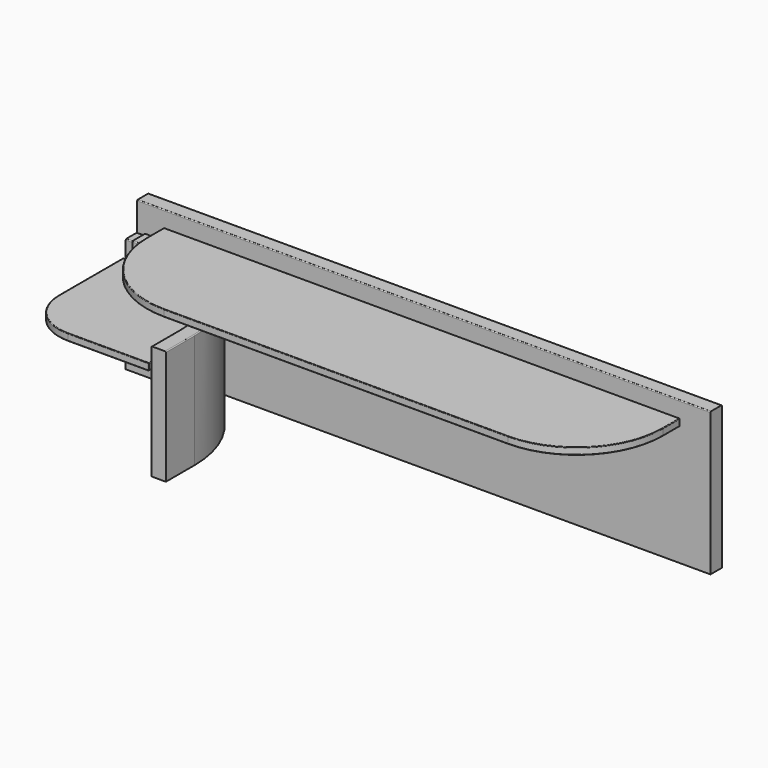
from build123d import *

# Parameters (mm, degrees)
F0_W                      = 2000
F0_H                      = 50
F1_DEPTH                  = 500
F4_DEPTH                  = 24
F5_R                      = 3
F6_R                      = 2
F8_DEPTH                  = 400
F11_DEPTH                 = 35
F13_DEPTH                 = 24
F14_R                     = 7.5
F15_DEPTH                 = 10
DRAFT_F15_DRAFTED_ANGLE   = 45
DRAFT_F15_2_DRAFTED_ANGLE = 45
F16_R                     = 5
F17_DEPTH                 = 6
F18_R                     = 3.5
F19_DEPTH                 = 25
F20_R                     = 3
F21_R                     = 2


# Not quite as in the source:
# - an extrude with a draft is written as a straight extrude whose walls are then drafted


with BuildPart() as f1:
    # F0 (on Top) → F1 (new body)
    with BuildSketch(Plane.XY):
        with Locations((1000, 25)):
            Rectangle(F0_W, F0_H)
    extrude(amount=F1_DEPTH)

    # F5
    f5_edges = [f1.edges().sort_by_distance(p)[0] for p in [
        (1000, 0, 500),
        (1000, 50, 500),
    ]]
    fillet(f5_edges, radius=F5_R)


with BuildPart() as f4:
    # F3 (on offset) → F4 (new body)
    with BuildSketch(Plane.XY.offset(426)):
        with BuildLine():
            Line((1900, -8), (100, -8))
            Line((100, -8), (100, -83))
            ThreePointArc((100, -83), (187.867965644, -295.132034356), (400, -383))
            Line((400, -383), (1600, -383))
            ThreePointArc((1600, -383), (1812.132034356, -295.132034356), (1900, -83))
            Line((1900, -83), (1900, -8))
        make_face()
    extrude(amount=F4_DEPTH)

    # F6
    f6_edges = [f4.edges().sort_by_distance(p)[0] for p in [
        (100, -45.5, 450),
        (187.867966, -295.132034, 450),
        (1000, -383, 426),
        (100, -8, 438),
        (1000, -8, 450),
        (1000, -8, 426),
        (1900, -8, 438),
    ]]
    fillet(f6_edges, radius=F6_R)


with BuildPart() as f8:
    # F7 (on Top) → F8 (new body)
    with BuildSketch(Plane.XY):
        with BuildLine():
            Line((125, 0), (0, 0))
            Line((0, 0), (0, -50))
            Line((0, -50), (125, -50))
            ThreePointArc((125, -50), (354.8097038856, -145.1902961144), (450, -375))
            Line((450, -375), (450, -500))
            Line((450, -500), (500, -500))
            Line((500, -500), (500, -375))
            ThreePointArc((500, -375), (390.165042945, -109.834957055), (125, 0))
        make_face()
    extrude(amount=F8_DEPTH)

    # F20
    f20_edges = [f8.edges().sort_by_distance(p)[0] for p in [
        (354.809704, -145.190296, 400),
        (62.5, 0, 400),
        (450, -437.5, 400),
        (500, -437.5, 400),
        (390.165043, -109.834957, 400),
        (62.5, -50, 400),
    ]]
    fillet(f20_edges, radius=F20_R)


with BuildPart() as f11:
    # F10 (on offset) → F11 (new body, symmetric)
    with BuildSketch(Plane(origin=(62.5, 0, 0), x_dir=(0, -1, 0), z_dir=(-1, 0, 0))):
        with BuildLine():
            ThreePointArc((50, 319), (50.8786796564, 316.8786796564), (53, 316))
            Line((53, 316), (104, 316))
            ThreePointArc((104, 316), (104.7071067812, 316.2928932188), (105, 317))
            Line((105, 317), (105, 320))
            ThreePointArc((105, 320), (104.7071067812, 320.7071067812), (104, 321))
            Line((104, 321), (58, 321))
            ThreePointArc((58, 321), (55.8786796564, 321.8786796564), (55, 324))
            Line((55, 324), (55, 402))
            ThreePointArc((55, 402), (54.1213203436, 404.1213203436), (52, 405))
            Line((52, 405), (-2, 405))
            ThreePointArc((-2, 405), (-4.1213203436, 404.1213203436), (-5, 402))
            Line((-5, 402), (-5, 355))
            ThreePointArc((-5, 355), (-1.4644660941, 353.5355339059), (0, 350))
            Line((0, 350), (0, 397))
            ThreePointArc((0, 397), (0.8786796564, 399.1213203436), (3, 400))
            Line((3, 400), (47, 400))
            ThreePointArc((47, 400), (49.1213203436, 399.1213203436), (50, 397))
            Line((50, 397), (50, 319))
        make_face()
        with BuildLine():
            ThreePointArc((-5, 345), (-1.4644660941, 346.4644660941), (0, 350))
            ThreePointArc((0, 350), (-1.4644660941, 353.5355339059), (-5, 355))
            Line((-5, 355), (-5, 345))
        make_face()
        with BuildLine():
            ThreePointArc((-5, 355), (-10, 350), (-5, 345))
            Line((-5, 345), (-5, 355))
        make_face()
    extrude(amount=F11_DEPTH, both=True)


with BuildPart() as f13:
    # F12 (on face) → F13 (new body)
    with BuildSketch(Plane.XY.offset(321)):
        with BuildLine():
            Line((125, -60), (-1.2988302449, -60))
            Line((-1.2988302449, -60), (-1.2988302449, -340))
            ThreePointArc((-1.2988302449, -340), (45.5640847653, -453.1370849898), (158.7011697551, -500))
            Line((158.7011697551, -500), (440, -500))
            Line((440, -500), (440, -375))
            ThreePointArc((440, -375), (347.7386360738, -152.2613639262), (125, -60))
        make_face()
    extrude(amount=F13_DEPTH)


with BuildPart() as f15_drafted:
    # F14 (on face) → F15 (new body)
    with BuildSketch(Plane(origin=(0, 0, 316), x_dir=(1, 0, 0), z_dir=(0, 0, -1))):
        with Locations((47.5, 82)):
            Circle(F14_R)
    extrude(amount=-F15_DEPTH)

    # draft_F15_drafted
    draft_f15_drafted_walls = [f15_drafted.faces().sort_by_distance(p)[0] for p in [
        (40, -82, 322.6666666667),
    ]]
    draft(draft_f15_drafted_walls, neutral_plane=Plane.XY.offset(316), angle=DRAFT_F15_DRAFTED_ANGLE)


with BuildPart() as f11_1:
    add(f11.part)

    # join_F15_drafted: cut F15_drafted
    add(f15_drafted.part, mode=Mode.SUBTRACT)


with BuildPart() as f13_1:
    add(f13.part)

    # join_F15_drafted: cut F15_drafted
    add(f15_drafted.part, mode=Mode.SUBTRACT)


with BuildPart() as f15_2_drafted:
    # F14 (on face) → F15, piece 2 (new body)
    with BuildSketch(Plane(origin=(0, 0, 316), x_dir=(1, 0, 0), z_dir=(0, 0, -1))):
        with Locations((77.5, 82)):
            Circle(F14_R)
    extrude(amount=-F15_DEPTH)

    # draft_F15_2_drafted
    draft_f15_2_drafted_walls = [f15_2_drafted.faces().sort_by_distance(p)[0] for p in [
        (70, -82, 322.6666666667),
    ]]
    draft(draft_f15_2_drafted_walls, neutral_plane=Plane.XY.offset(316), angle=DRAFT_F15_2_DRAFTED_ANGLE)


with BuildPart() as f11_2:
    add(f11_1.part)

    # join_F15_2_drafted: cut F15_2_drafted
    add(f15_2_drafted.part, mode=Mode.SUBTRACT)


with BuildPart() as f13_2:
    add(f13_1.part)

    # join_F15_2_drafted: cut F15_2_drafted
    add(f15_2_drafted.part, mode=Mode.SUBTRACT)

    # F16 (on face) → F17 (cut)
    with BuildSketch(Plane(origin=(0, 0, 316), x_dir=(1, 0, 0), z_dir=(0, 0, -1))):
        with Locations((47.5, 82)):
            Circle(F16_R)
        with Locations((77.5, 82)):
            Circle(F16_R)
        with Locations((416.8352910245, 422.8001448106)):
            Circle(F16_R)
        with Locations((416.7060655573, 452.7998664889)):
            Circle(F16_R)
    extrude(amount=-F17_DEPTH, mode=Mode.SUBTRACT)

    # F18 (on face) → F19 (cut)
    with BuildSketch(Plane(origin=(0, 0, 316), x_dir=(1, 0, 0), z_dir=(0, 0, -1))):
        with Locations((47.5, 82)):
            Circle(F18_R)
        with Locations((77.5, 82)):
            Circle(F18_R)
        with Locations((416.8352910245, 422.8001448106)):
            Circle(F18_R)
        with Locations((416.7060655573, 452.7998664889)):
            Circle(F18_R)
    extrude(amount=-F19_DEPTH, mode=Mode.SUBTRACT)

    # F21
    f21_edges = [f13_2.edges().sort_by_distance(p)[0] for p in [
        (-1.29883, -200, 345),
        (-1.29883, -200, 321),
        (-1.29883, -60, 333),
        (61.850585, -60, 345),
        (61.850585, -60, 321),
        (440, -500, 333),
        (347.738636, -152.261364, 321),
        (347.738636, -152.261364, 345),
        (440, -437.5, 321),
        (45.564085, -453.137085, 321),
        (299.350585, -500, 321),
        (45.564085, -453.137085, 345),
        (299.350585, -500, 345),
        (440, -437.5, 345),
    ]]
    fillet(f21_edges, radius=F21_R)


solid = Compound([f1.part, f4.part, f8.part, f11_2.part, f13_2.part])
